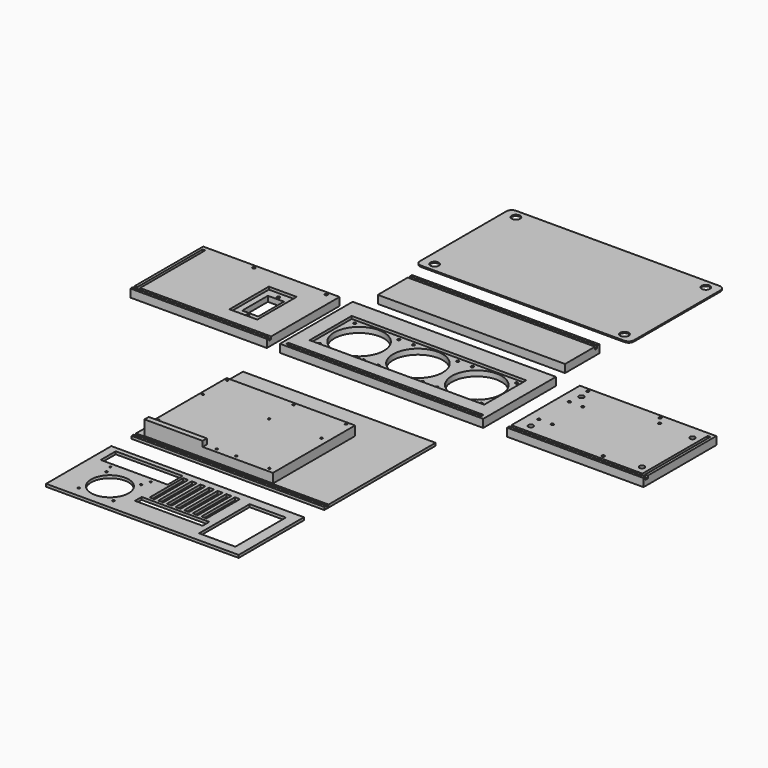
from build123d import *

# Parameters (mm, degrees)
F0_W      = 482.6
F0_H      = 215.9
F0_W_2    = 463.55
F0_H_2    = 6.4
F0_W_3    = 414.33164
F0_H_3    = 125
F0_R      = 3.1877
F0_R_2    = 59
F1_DEPTH  = 12.7
F2_DEPTH  = 6.35
F3_R      = 6
F3_R_2    = 3.302
F3_W      = 323.85
F3_H      = 6.35
F3_W_2    = 6.3754
F3_H_2    = 2.7085937142
F3_H_3    = 193.625
F4_DEPTH  = 12.7
F5_DEPTH  = 6.35
F6_R      = 3.302
F6_W      = 66.04
F6_H      = 116.84
F6_W_2    = 38.1
F6_H_2    = 76.2
F6_W_3    = 323.85
F6_H_3    = 6.35
F6_W_4    = 6.3754
F6_H_4    = 193.625
F6_H_5    = 3.846908319
F7_DEPTH  = 12.7
F8_DEPTH  = 6.35
F9_DEPTH  = 6.35
F10_R     = 2.5
F10_W     = 138.0889187211
F10_H     = 12.6182494217
F11_DEPTH = 25.4
F12_DEPTH = 38.1
F13_W     = 457.2
F13_H     = 317.4746
F13_H_2   = 6.3754
F13_H_3   = 6.35
F14_DEPTH = 3.2
F15_DEPTH = 3.2
F16_W     = 457.2
F16_H     = 193.6500064
F16_R     = 2.5
F16_R_2   = 44.5
F16_W_2   = 160.4000098
F16_H_2   = 20
F16_R_3   = 2.0970704069
F16_R_4   = 2.1817303996
F16_W_3   = 12.0000014
F16_H_3   = 99.38
F16_W_4   = 158.75
F16_H_4   = 44.45
F16_W_5   = 86
F16_H_5   = 150
F17_DEPTH = 6.3754
F18_W     = 444.5
F18_H     = 88.8746
F18_H_2   = 6.3754
F18_H_3   = 6.35
F19_DEPTH = 12.7
F20_DEPTH = 6.35
F21_R     = 10
F22_DEPTH = 3


# Not quite as in the source:
# - a feature names something its author has since deleted; it is built from what else it names


with BuildPart() as f1:
    # F0 (on Top) → F1 (new body)
    with BuildSketch(Plane.XY):
        Rectangle(F0_W, F0_H)
        with Locations((0, -98.4)):
            Rectangle(F0_W_2, F0_H_2, mode=Mode.SUBTRACT)
        Rectangle(F0_W_3, F0_H_3, mode=Mode.SUBTRACT)
        Rectangle(F0_W_3, F0_H_3)
        with Locations((-192.2, -52.5)):
            Circle(F0_R, mode=Mode.SUBTRACT)
        with Locations((-87.2, -52.5)):
            Circle(F0_R, mode=Mode.SUBTRACT)
        with Locations((-52.5, -52.5)):
            Circle(F0_R, mode=Mode.SUBTRACT)
        with Locations((52.5, -52.5)):
            Circle(F0_R, mode=Mode.SUBTRACT)
        with Locations((87.2, -52.5)):
            Circle(F0_R, mode=Mode.SUBTRACT)
        with Locations((192.2, -52.5)):
            Circle(F0_R, mode=Mode.SUBTRACT)
        with Locations((-139.7, 0)):
            Circle(F0_R_2, mode=Mode.SUBTRACT)
        with Locations((-192.2, 52.5)):
            Circle(F0_R, mode=Mode.SUBTRACT)
        with Locations((-87.2, 52.5)):
            Circle(F0_R, mode=Mode.SUBTRACT)
        with Locations((-52.5, 52.5)):
            Circle(F0_R, mode=Mode.SUBTRACT)
        Circle(F0_R_2, mode=Mode.SUBTRACT)
        with Locations((52.5, 52.5)):
            Circle(F0_R, mode=Mode.SUBTRACT)
        with Locations((87.2, 52.5)):
            Circle(F0_R, mode=Mode.SUBTRACT)
        with Locations((139.7, 0)):
            Circle(F0_R_2, mode=Mode.SUBTRACT)
        with Locations((192.2, 52.5)):
            Circle(F0_R, mode=Mode.SUBTRACT)
        with Locations((0, -98.4)):
            Rectangle(F0_W_2, F0_H_2)
    extrude(amount=-F1_DEPTH)

    # F0 (on Top) → F2 (join)
    with BuildSketch(Plane.XY):
        Rectangle(F0_W, F0_H)
        with Locations((0, -98.4)):
            Rectangle(F0_W_2, F0_H_2, mode=Mode.SUBTRACT)
        Rectangle(F0_W_3, F0_H_3, mode=Mode.SUBTRACT)
    extrude(amount=F2_DEPTH)


with BuildPart() as f4:
    # F3 (on Top) → F4 (new body)
    with BuildSketch(Plane.XY):
        Polygon((298.0011743546, 107.95), (298.0011743546, -95.2), (609.1257743546, -95.2), (609.1257743546, 98.425), (615.5011743546, 98.425), (615.5011743546, -95.2), (621.8511743546, -95.2), (621.8511743546, 107.95), align=None)
        with Locations((328.0011743546, -74.95)):
            Circle(F3_R, mode=Mode.SUBTRACT)
        with BuildLine():
            Line((351.8992377546, -45.0850025), (326.7031743546, -45.0850025))
            ThreePointArc((326.7031743546, -45.0850025), (321.0663077631, -47.4198690915), (323.4011743546, -41.7830025))
            Line((323.4011743546, -41.7830025), (323.4011743546, 41.7829975))
            ThreePointArc((323.4011743546, 41.7829975), (321.0663077631, 47.4198640915), (326.7031743546, 45.0849975))
            Line((326.7031743546, 45.0849975), (351.8992377546, 45.0849975))
            ThreePointArc((351.8992377546, 45.0849975), (355.2012377546, 48.3869975), (358.5032377546, 45.0849975))
            ThreePointArc((358.5032377546, 45.0849975), (357.536104346, 42.7501309085), (355.2012377546, 41.7829975))
            Line((355.2012377546, 41.7829975), (355.2012377546, -41.7830025))
            ThreePointArc((355.2012377546, -41.7830025), (357.536104346, -42.7501359085), (358.5032377546, -45.0850025))
            ThreePointArc((358.5032377546, -45.0850025), (355.2012377546, -48.3870025), (351.8992377546, -45.0850025))
        make_face(mode=Mode.SUBTRACT)
        with Locations((508.1257743546, -85.4085937142)):
            Circle(F3_R_2, mode=Mode.SUBTRACT)
        with Locations((591.8511743546, -74.95)):
            Circle(F3_R, mode=Mode.SUBTRACT)
        with Locations((328.0011743546, 74.95)):
            Circle(F3_R, mode=Mode.SUBTRACT)
        with Locations((323.4011743546, 99.95)):
            Circle(F3_R_2, mode=Mode.SUBTRACT)
        with Locations((494.8511743546, 99.95)):
            Circle(F3_R_2, mode=Mode.SUBTRACT)
        with Locations((508.1257743546, 81.95)):
            Circle(F3_R_2, mode=Mode.SUBTRACT)
        with Locations((591.8511743546, 74.95)):
            Circle(F3_R, mode=Mode.SUBTRACT)
        Polygon((298.0011743546, -95.2), (298.0011743546, -101.6), (621.8511743546, -101.6), (621.8511743546, -95.2), (615.5011743546, -95.2), (615.5011743546, -97.9085937142), (609.1257743546, -97.9085937142), (609.1257743546, -95.2), align=None)
        with Locations((459.9261743546, -104.775)):
            Rectangle(F3_W, F3_H)
        with Locations((612.3134743546, -96.5542968571)):
            Rectangle(F3_W_2, F3_H_2)
        with Locations((612.3134743546, 1.6125)):
            Rectangle(F3_W_2, F3_H_3)
        with Locations((328.0011743546, 74.95)):
            Circle(F3_R)
        with Locations((328.0011743546, 74.95)):
            Circle(F3_R_2, mode=Mode.SUBTRACT)
        with Locations((328.0011743546, -74.95)):
            Circle(F3_R)
        with Locations((328.0011743546, -74.95)):
            Circle(F3_R_2, mode=Mode.SUBTRACT)
        with Locations((591.8511743546, -74.95)):
            Circle(F3_R)
        with Locations((591.8511743546, -74.95)):
            Circle(F3_R_2, mode=Mode.SUBTRACT)
        with Locations((591.8511743546, 74.95)):
            Circle(F3_R)
        with Locations((591.8511743546, 74.95)):
            Circle(F3_R_2, mode=Mode.SUBTRACT)
        with BuildLine():
            ThreePointArc((323.4011743546, -41.7830025), (325.736040946, -42.7501359085), (326.7031743546, -45.0850025))
            Line((326.7031743546, -45.0850025), (351.8992377546, -45.0850025))
            ThreePointArc((351.8992377546, -45.0850025), (352.8663711631, -42.7501359085), (355.2012377546, -41.7830025))
            Line((355.2012377546, -41.7830025), (355.2012377546, 41.7829975))
            ThreePointArc((355.2012377546, 41.7829975), (352.8663711631, 42.7501309085), (351.8992377546, 45.0849975))
            Line((351.8992377546, 45.0849975), (326.7031743546, 45.0849975))
            ThreePointArc((326.7031743546, 45.0849975), (325.736040946, 42.7501309085), (323.4011743546, 41.7829975))
            Line((323.4011743546, 41.7829975), (323.4011743546, -41.7830025))
        make_face()
    extrude(amount=-F4_DEPTH)

    # F3 (on Top) → F5 (join)
    with BuildSketch(Plane.XY):
        Polygon((298.0011743546, 107.95), (298.0011743546, -95.2), (609.1257743546, -95.2), (609.1257743546, 98.425), (615.5011743546, 98.425), (615.5011743546, -95.2), (621.8511743546, -95.2), (621.8511743546, 107.95), align=None)
        with Locations((328.0011743546, -74.95)):
            Circle(F3_R, mode=Mode.SUBTRACT)
        with BuildLine():
            Line((351.8992377546, -45.0850025), (326.7031743546, -45.0850025))
            ThreePointArc((326.7031743546, -45.0850025), (321.0663077631, -47.4198690915), (323.4011743546, -41.7830025))
            Line((323.4011743546, -41.7830025), (323.4011743546, 41.7829975))
            ThreePointArc((323.4011743546, 41.7829975), (321.0663077631, 47.4198640915), (326.7031743546, 45.0849975))
            Line((326.7031743546, 45.0849975), (351.8992377546, 45.0849975))
            ThreePointArc((351.8992377546, 45.0849975), (355.2012377546, 48.3869975), (358.5032377546, 45.0849975))
            ThreePointArc((358.5032377546, 45.0849975), (357.536104346, 42.7501309085), (355.2012377546, 41.7829975))
            Line((355.2012377546, 41.7829975), (355.2012377546, -41.7830025))
            ThreePointArc((355.2012377546, -41.7830025), (357.536104346, -42.7501359085), (358.5032377546, -45.0850025))
            ThreePointArc((358.5032377546, -45.0850025), (355.2012377546, -48.3870025), (351.8992377546, -45.0850025))
        make_face(mode=Mode.SUBTRACT)
        with Locations((508.1257743546, -85.4085937142)):
            Circle(F3_R_2, mode=Mode.SUBTRACT)
        with Locations((591.8511743546, -74.95)):
            Circle(F3_R, mode=Mode.SUBTRACT)
        with Locations((328.0011743546, 74.95)):
            Circle(F3_R, mode=Mode.SUBTRACT)
        with Locations((323.4011743546, 99.95)):
            Circle(F3_R_2, mode=Mode.SUBTRACT)
        with Locations((494.8511743546, 99.95)):
            Circle(F3_R_2, mode=Mode.SUBTRACT)
        with Locations((508.1257743546, 81.95)):
            Circle(F3_R_2, mode=Mode.SUBTRACT)
        with Locations((591.8511743546, 74.95)):
            Circle(F3_R, mode=Mode.SUBTRACT)
        with Locations((459.9261743546, -104.775)):
            Rectangle(F3_W, F3_H)
        with BuildLine():
            ThreePointArc((323.4011743546, -41.7830025), (325.736040946, -42.7501359085), (326.7031743546, -45.0850025))
            Line((326.7031743546, -45.0850025), (351.8992377546, -45.0850025))
            ThreePointArc((351.8992377546, -45.0850025), (352.8663711631, -42.7501359085), (355.2012377546, -41.7830025))
            Line((355.2012377546, -41.7830025), (355.2012377546, 41.7829975))
            ThreePointArc((355.2012377546, 41.7829975), (352.8663711631, 42.7501309085), (351.8992377546, 45.0849975))
            Line((351.8992377546, 45.0849975), (326.7031743546, 45.0849975))
            ThreePointArc((326.7031743546, 45.0849975), (325.736040946, 42.7501309085), (323.4011743546, 41.7829975))
            Line((323.4011743546, 41.7829975), (323.4011743546, -41.7830025))
        make_face()
    extrude(amount=F5_DEPTH)


with BuildPart() as f7:
    # F6 (on Top) → F7 (new body)
    with BuildSketch(Plane.XY):
        Polygon((-272.3593753815, -95.2), (-272.3593753815, 107.95), (-596.2093753815, 107.95), (-596.2093753815, -95.2), (-589.8593753815, -95.2), (-589.8593753815, 98.425), (-583.4839753815, 98.425), (-583.4839753815, -95.2), align=None)
        with Locations((-469.2093753815, 99.95)):
            Circle(F6_R, mode=Mode.SUBTRACT)
        with Locations((-367.6093753815, 0)):
            Rectangle(F6_W, F6_H, mode=Mode.SUBTRACT)
        with Locations((-297.7593753815, 99.95)):
            Circle(F6_R, mode=Mode.SUBTRACT)
        with Locations((-367.6093753815, 0)):
            Rectangle(F6_W, F6_H)
        with Locations((-367.6093753815, -45.6)):
            Circle(F6_R, mode=Mode.SUBTRACT)
        with Locations((-367.6093753815, 0)):
            Rectangle(F6_W_2, F6_H_2, mode=Mode.SUBTRACT)
        with Locations((-367.6093753815, 45.6)):
            Circle(F6_R, mode=Mode.SUBTRACT)
        with Locations((-434.2843753815, -104.775)):
            Rectangle(F6_W_3, F6_H_3)
        Polygon((-272.3593753815, -101.6), (-272.3593753815, -95.2), (-583.4839753815, -95.2), (-583.4839753815, -99.046908319), (-589.8593753815, -99.046908319), (-589.8593753815, -95.2), (-596.2093753815, -95.2), (-596.2093753815, -101.6), align=None)
        with Locations((-586.6716753815, 1.6125)):
            Rectangle(F6_W_4, F6_H_4)
        with Locations((-586.6716753815, -97.1234541595)):
            Rectangle(F6_W_4, F6_H_5)
    extrude(amount=-F7_DEPTH)

    # F6 (on Top) → F8 (join)
    with BuildSketch(Plane.XY):
        Polygon((-272.3593753815, -95.2), (-272.3593753815, 107.95), (-596.2093753815, 107.95), (-596.2093753815, -95.2), (-589.8593753815, -95.2), (-589.8593753815, 98.425), (-583.4839753815, 98.425), (-583.4839753815, -95.2), align=None)
        with Locations((-469.2093753815, 99.95)):
            Circle(F6_R, mode=Mode.SUBTRACT)
        with Locations((-367.6093753815, 0)):
            Rectangle(F6_W, F6_H, mode=Mode.SUBTRACT)
        with Locations((-297.7593753815, 99.95)):
            Circle(F6_R, mode=Mode.SUBTRACT)
        with Locations((-367.6093753815, 0)):
            Rectangle(F6_W, F6_H)
        with Locations((-367.6093753815, -45.6)):
            Circle(F6_R, mode=Mode.SUBTRACT)
        with Locations((-367.6093753815, 0)):
            Rectangle(F6_W_2, F6_H_2, mode=Mode.SUBTRACT)
        with Locations((-367.6093753815, 45.6)):
            Circle(F6_R, mode=Mode.SUBTRACT)
        with Locations((-434.2843753815, -104.775)):
            Rectangle(F6_W_3, F6_H_3)
    extrude(amount=F8_DEPTH)

    # F6 (on Top) → F9 (cut)
    with BuildSketch(Plane.XY):
        with Locations((-367.6093753815, 0)):
            Rectangle(F6_W, F6_H)
        with Locations((-367.6093753815, -45.6)):
            Circle(F6_R, mode=Mode.SUBTRACT)
        with Locations((-367.6093753815, 0)):
            Rectangle(F6_W_2, F6_H_2, mode=Mode.SUBTRACT)
        with Locations((-367.6093753815, 45.6)):
            Circle(F6_R, mode=Mode.SUBTRACT)
    extrude(amount=F9_DEPTH, mode=Mode.SUBTRACT)


with BuildPart() as f11:
    # F10 (on Top) → F11 (new body)
    with BuildSketch(Plane.XY):
        Polygon((95.25, -549.4468963333), (95.25, -305.6068963333), (-209.55, -305.6068963333), (-209.55, -536.8286469116), (-71.4610812789, -536.8286469116), (-71.4610812789, -549.4468963333), align=None)
        with Locations((-203.2, -516.4268963333)):
            Circle(F10_R, mode=Mode.SUBTRACT)
        with Locations((-45.72, -539.2868963333)):
            Circle(F10_R, mode=Mode.SUBTRACT)
        with Locations((0, -539.2868963333)):
            Circle(F10_R, mode=Mode.SUBTRACT)
        with Locations((78.74, -539.2868963333)):
            Circle(F10_R, mode=Mode.SUBTRACT)
        with Locations((-203.2, -384.3468963333)):
            Circle(F10_R, mode=Mode.SUBTRACT)
        with Locations((-203.2, -311.9568963333)):
            Circle(F10_R, mode=Mode.SUBTRACT)
        with Locations((-45.72, -384.3468963333)):
            Circle(F10_R, mode=Mode.SUBTRACT)
        with Locations((78.74, -384.3468963333)):
            Circle(F10_R, mode=Mode.SUBTRACT)
        with Locations((-45.72, -311.9568963333)):
            Circle(F10_R, mode=Mode.SUBTRACT)
        with Locations((78.74, -311.9568963333)):
            Circle(F10_R, mode=Mode.SUBTRACT)
        with Locations((-140.5055406395, -543.1377716225)):
            Rectangle(F10_W, F10_H)
    extrude(amount=F11_DEPTH)

    # F10 (on Top) → F12 (join)
    with BuildSketch(Plane.XY):
        with Locations((-140.5055406395, -543.1377716225)):
            Rectangle(F10_W, F10_H)
    extrude(amount=F12_DEPTH)


with BuildPart() as f14:
    # F13 (on Top) → F14 (new body)
    with BuildSketch(Plane.XY):
        with Locations((0, -392.2095963333)):
            Rectangle(F13_W, F13_H)
        with Locations((0, -554.1345963333)):
            Rectangle(F13_W, F13_H_2)
        with Locations((0, -560.4972963333)):
            Rectangle(F13_W, F13_H_3)
    extrude(amount=-F14_DEPTH)

    # F13 (on Top) → F15 (join)
    with BuildSketch(Plane.XY):
        with Locations((0, -392.2095963333)):
            Rectangle(F13_W, F13_H)
        with Locations((0, -560.4972963333)):
            Rectangle(F13_W, F13_H_3)
    extrude(amount=F15_DEPTH)


with BuildPart() as f17:
    # F16 (on Top) → F17 (new body)
    with BuildSketch(Plane.XY):
        with Locations((0, -720.8472931333)):
            Rectangle(F16_W, F16_H)
        with Locations((-171.0694, -792.8822963333)):
            Circle(F16_R, mode=Mode.SUBTRACT)
        with Locations((-88.5694, -792.8822963333)):
            Circle(F16_R, mode=Mode.SUBTRACT)
        with Locations((-129.8194, -751.6322963333)):
            Circle(F16_R_2, mode=Mode.SUBTRACT)
        with Locations((23.04998076, -758.2222783933)):
            Rectangle(F16_W_2, F16_H_2, mode=Mode.SUBTRACT)
        with Locations((-171.0694, -710.3822963333)):
            Circle(F16_R, mode=Mode.SUBTRACT)
        with Locations((-177.92501754, -690.1722947933)):
            Circle(F16_R_3, mode=Mode.SUBTRACT)
        with Locations((-88.5694, -710.3822963333)):
            Circle(F16_R, mode=Mode.SUBTRACT)
        with Locations((-81.72500674, -690.1722947933)):
            Circle(F16_R_4, mode=Mode.SUBTRACT)
        with Locations((-38.45002344, -690.9122783933)):
            Rectangle(F16_W_3, F16_H_3, mode=Mode.SUBTRACT)
        with Locations((-17.95002204, -690.9122783933)):
            Rectangle(F16_W_3, F16_H_3, mode=Mode.SUBTRACT)
        with Locations((-129.82501214, -657.4472903933)):
            Rectangle(F16_W_4, F16_H_4, mode=Mode.SUBTRACT)
        with Locations((2.54997936, -690.9122783933)):
            Rectangle(F16_W_3, F16_H_3, mode=Mode.SUBTRACT)
        with Locations((23.04998076, -690.9122783933)):
            Rectangle(F16_W_3, F16_H_3, mode=Mode.SUBTRACT)
        with Locations((43.54998216, -690.9122783933)):
            Rectangle(F16_W_3, F16_H_3, mode=Mode.SUBTRACT)
        with Locations((64.04998356, -690.9122783933)):
            Rectangle(F16_W_3, F16_H_3, mode=Mode.SUBTRACT)
        with Locations((84.54998496, -690.9122783933)):
            Rectangle(F16_W_3, F16_H_3, mode=Mode.SUBTRACT)
        with Locations((160.2, -720.8472931333)):
            Rectangle(F16_W_5, F16_H_5, mode=Mode.SUBTRACT)
    extrude(amount=F17_DEPTH)


with BuildPart() as f19:
    # F18 (on Top) → F19 (new body)
    with BuildSketch(Plane.XY):
        with Locations((0, 203.1873)):
            Rectangle(F18_W, F18_H)
        with Locations((0, 250.8123)):
            Rectangle(F18_W, F18_H_2)
        with Locations((0, 257.175)):
            Rectangle(F18_W, F18_H_3)
    extrude(amount=-F19_DEPTH)

    # F18 (on Top) → F20 (join)
    with BuildSketch(Plane.XY):
        with Locations((0, 257.175)):
            Rectangle(F18_W, F18_H_3)
        with Locations((0, 203.1873)):
            Rectangle(F18_W, F18_H)
    extrude(amount=F20_DEPTH)


with BuildPart() as f22:
    # F21 (on Top) → F22 (new body)
    with BuildSketch(Plane.XY):
        with BuildLine():
            ThreePointArc((-249.73, 318.2267664064), (-246.0102561211, 309.2465102853), (-237.03, 305.5267664064))
            Line((-237.03, 305.5267664064), (245.57, 305.5267664064))
            ThreePointArc((245.57, 305.5267664064), (254.5502561211, 309.2465102853), (258.27, 318.2267664064))
            Line((258.27, 318.2267664064), (258.27, 574.7667664064))
            ThreePointArc((258.27, 574.7667664064), (254.5502561211, 583.7470225275), (245.57, 587.4667664064))
            Line((245.57, 587.4667664064), (-237.03, 587.4667664064))
            ThreePointArc((-237.03, 587.4667664064), (-246.0102561211, 583.7470225275), (-249.73, 574.7667664064))
            Line((-249.73, 574.7667664064), (-249.73, 318.2267664064))
        make_face()
        with Locations((-221.0799938, 325.8467664064)):
            Circle(F21_R, mode=Mode.SUBTRACT)
        with Locations((229.6200062, 325.8467664064)):
            Circle(F21_R, mode=Mode.SUBTRACT)
        with Locations((-221.0799938, 567.1467664064)):
            Circle(F21_R, mode=Mode.SUBTRACT)
        with Locations((229.6200062, 567.1467664064)):
            Circle(F21_R, mode=Mode.SUBTRACT)
    extrude(amount=F22_DEPTH)


solid = Compound([f1.part, f4.part, f7.part, f11.part, f14.part, f17.part, f19.part, f22.part])
